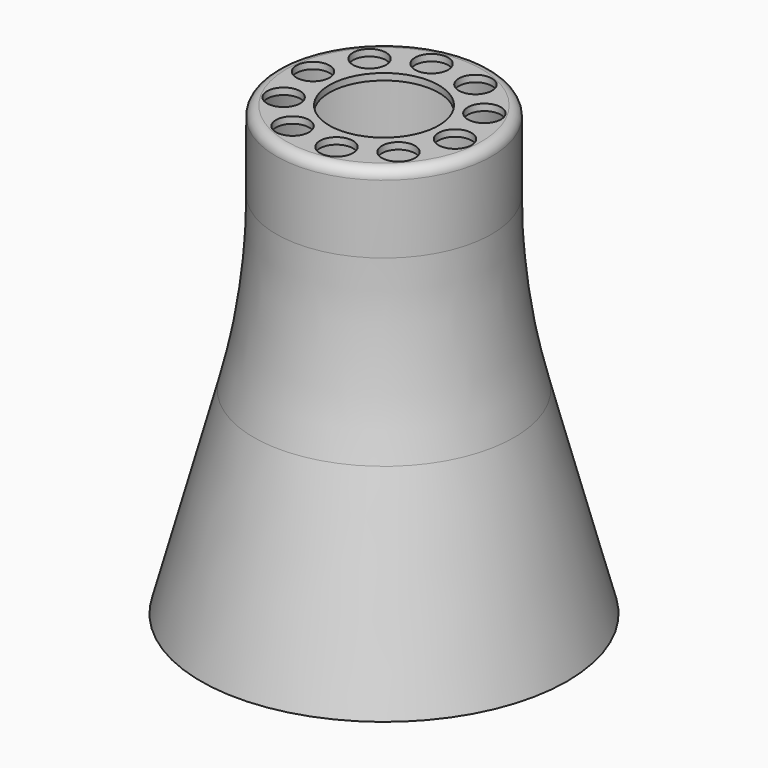
from build123d import *

# Parameters (mm, degrees)
F2_R            = 3
F3_R            = 200
F5_D            = 10
F5_COPIES_COUNT = 10


# Not quite as in the source:
# - a pattern or mirror of a feature is missing from the dataset's text; its kind, count and spacing are read off the source's solid


with BuildPart() as f1:
    # F0 (on Front) → F1 (revolve)
    with BuildSketch(Plane.XZ):
        Polygon((-16.5, 133), (-16.5, 135), (-32.5, 135), (-32.5, 85), (-55.2756813566, 0), (-53.2051289958, 0), (-30.5, 84.7366950048), (-30.5, 133), align=None)
    revolve(axis=Axis((0, 0, 82.1189115205), (0, 0, -1)))

    # F2
    f2_edges = [f1.edges().sort_by_distance(p)[0] for p in [
        (32.5, 0, 135),
    ]]
    fillet(f2_edges, radius=F2_R)

    # F3
    f3_edges = [f1.edges().sort_by_distance(p)[0] for p in [
        (32.5, 0, 85),
    ]]
    fillet(f3_edges, radius=F3_R)

    # F5 (through all)
    with Locations(Plane.XY.offset(135)):
        with Locations((-10.2066846848, -21.7215005869)):
            f5 = Hole(F5_D / 2)

    # F5_copies: F5 ×10 about axis
    f5_copies_axis = Axis((0, 0, 0), (0, 0, 1))
    for i in range(1, F5_COPIES_COUNT):
        add(f5.rotate(f5_copies_axis, i * 360 / F5_COPIES_COUNT), mode=Mode.SUBTRACT)


solid = f1.part
